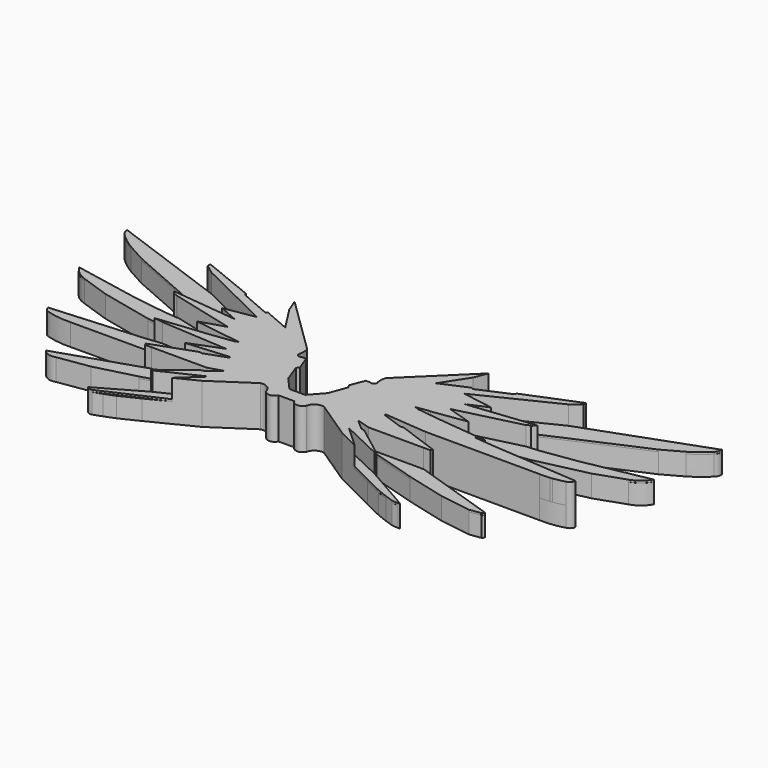
from build123d import *

# Parameters (mm, degrees)
F1_DEPTH = 5.08
F3_DEPTH = 0.508
F4_DEPTH = 5.334


# Not quite as in the source:
# - a feature names something its author has since deleted; it is built from what else it names


with BuildPart() as f1:
    # F0 (on Top) → F1 (new body)
    with BuildSketch(Plane.XY):
        with BuildLine():
            Line((-48.1556859188, 20.4166518488), (-45.7547713604, 18.6155719344))
            Line((-45.7547713604, 18.6155719344), (-76.2, 29.6858626598))
            ThreePointArc((-76.2, 29.6858626598), (-76.0861543316, 28.7560173531), (-75.5575876457, 27.9825896648))
            ThreePointArc((-75.5575876457, 27.9825896648), (-73.4489543022, 26.1296903536), (-71.1370066464, 24.5376889491))
            Line((-71.1370066464, 24.5376889491), (-66.2742528397, 21.8479481701))
            Line((-66.2742528397, 21.8479481701), (-58.5624668218, 18.4708371441))
            Line((-58.5624668218, 18.4708371441), (-35.3622883709, 8.3111182061))
            Line((-35.3622883709, 8.3111182061), (-29.5045119496, 5.7459068148))
            Line((-29.5045119496, 5.7459068148), (-46.2756385592, 7.5718067148))
            Line((-46.2756385592, 7.5718067148), (-46.5527664405, 7.6019780791))
            Line((-46.5527664405, 7.6019780791), (-45.7425475216, 6.6796372943))
            ThreePointArc((-45.7425475216, 6.6796372943), (-45.1421148672, 6.5863049394), (-44.6164082899, 6.2815708004))
            Line((-44.6164082899, 6.2815708004), (-48.1919185541, 6.5892115587))
            Line((-48.1919185541, 6.5892115587), (-57.1823799566, 7.911566844))
            Line((-57.1823799566, 7.911566844), (-73.6501002366, 11.0943052422))
            ThreePointArc((-73.6501002366, 11.0943052422), (-71.9881572625, 9.0822772608), (-69.6750634505, 7.8740107076))
            Line((-69.6750634505, 7.8740107076), (-62.2713321356, 5.3338180736))
            Line((-62.2713321356, 5.3338180736), (-48.9967867739, 2.3219788609))
            Line((-48.9967867739, 2.3219788609), (-26.0691300337, -1.000935792))
            Line((-26.0691300337, -1.000935792), (-25.5777875701, -1.000935792))
            Line((-25.5777875701, -1.000935792), (-22.5801609633, -1.4353830401))
            Line((-22.5801609633, -1.4353830401), (-23.598120873, -1.8208819811))
            Line((-23.598120873, -1.8208819811), (-29.6029133803, -2.5945054753))
            Line((-29.6029133803, -2.5945054753), (-42.3688777231, -3.9362549145))
            Line((-42.3688777231, -3.9362549145), (-40.0474588237, -4.2726991035))
            Line((-40.0474588237, -4.2726991035), (-44.609626805, -4.752199607))
            Line((-44.609626805, -4.752199607), (-67.5607632512, -6.4104881929))
            ThreePointArc((-67.5607632512, -6.4104881929), (-67.1610869389, -7.3442465842), (-66.2705799276, -7.8327577416))
            ThreePointArc((-66.2705799276, -7.8327577416), (-63.2022368013, -8.4748868798), (-60.0694551881, -8.5877528823))
            Line((-60.0694551881, -8.5877528823), (-30.8294042942, -8.5236300949))
            Line((-30.8294042942, -8.5236300949), (-19.9096897181, -7.6185828777))
            Line((-19.9096897181, -7.6185828777), (-19.9096897181, -7.9501351804))
            Line((-19.9096897181, -7.9501351804), (-25.3987332293, -9.9026141464))
            Line((-25.3987332293, -9.9026141464), (-26.177360162, -9.7897674271))
            Line((-26.177360162, -9.7897674271), (-36.7820497354, -13.6233741381))
            Line((-36.7820497354, -13.6233741381), (-36.5863546909, -14.1647142792))
            Line((-36.5863546909, -14.1647142792), (-34.8660396089, -14.1609416661))
            Line((-34.8660396089, -14.1609416661), (-56.2699958177, -21.2122522245))
            ThreePointArc((-56.2699958177, -21.2122522245), (-54.7449311758, -22.2892299122), (-52.8788538396, -22.2304210928))
            Line((-52.8788538396, -22.2304210928), (-44.9235154086, -21.0280555311))
            Line((-44.9235154086, -21.0280555311), (-34.6822151602, -18.375633369))
            Line((-34.6822151602, -18.375633369), (-17.2204277187, -13.107625142))
            Line((-17.2204277187, -13.107625142), (-19.9096897181, -15.4653348387))
            Line((-19.9096897181, -15.4653348387), (-20.953229799, -15.7801581493))
            Line((-20.953229799, -15.7801581493), (-28.8616205932, -21.8016796487))
            Line((-28.8616205932, -21.8016796487), (-28.4234154154, -21.865188904))
            Line((-28.4234154154, -21.865188904), (-39.7813339224, -28.3391517425))
            ThreePointArc((-39.7813339224, -28.3391517425), (-39.1733915256, -28.7871689471), (-38.4182988766, -28.7749843229))
            Line((-38.4182988766, -28.7749843229), (-36.202970226, -27.9869813522))
            Line((-36.202970226, -27.9869813522), (-33.5857428013, -26.9761213966))
            Line((-33.5857428013, -26.9761213966), (-28.8616205932, -24.6837501383))
            Line((-28.8616205932, -24.6837501383), (-17.9108938238, -19.2006514725))
            Line((-17.9108938238, -19.2006514725), (-8.1309387585, -12.6873564961))
            ThreePointArc((-8.1309387585, -12.6873564961), (-6.2540728234, -13.0090484092), (-5.155673966, -14.5645648429))
            ThreePointArc((-5.155673966, -14.5645648429), (-3.5896736899, -15.5530124109), (-2.0236734137, -14.5645648429))
            Line((-2.0236734137, -14.5645648429), (-2.0236734137, -12.7489120778))
            Line((-2.0236734137, -12.7489120778), (-2.0236734137, -11.069433426))
            Line((-2.0236734137, -11.069433426), (-5.0648916394, -7.6650855824))
            Line((-5.0648916394, -7.6650855824), (-6.7443696679, -3.1259542931))
            Line((-6.7443696679, -3.1259542931), (-6.245065625, -2.3543018679))
            Line((-6.245065625, -2.3543018679), (-7.6521960504, 1.2770033506))
            Line((-7.6521960504, 1.2770033506), (-8.7869788728, 1.2770033506))
            ThreePointArc((-8.7869788728, 1.2770033506), (-9.7426169592, 1.3351185179), (-9.9217616951, 2.2756123714))
            ThreePointArc((-9.9217616951, 2.2756123714), (-9.8496747918, 3.482472458), (-10.0676489398, 4.6716717941))
            Line((-10.0676489398, 4.6716717941), (-24.8806389617, 19.145210523))
            Line((-24.8806389617, 19.145210523), (-23.5544247636, 15.7928414245))
            Line((-23.5544247636, 15.7928414245), (-19.3413656313, 9.2291376834))
            Line((-19.3413656313, 9.2291376834), (-26.048319795, 12.124898042))
            Line((-26.048319795, 12.124898042), (-26.5740321425, 11.8401364598))
            Line((-26.5740321425, 11.8401364598), (-34.4378306482, 15.2353700376))
            Line((-34.4378306482, 15.2353700376), (-34.7242604777, 15.8157629926))
            Line((-34.7242604777, 15.8157629926), (-48.1556859188, 21.2768864279))
            ThreePointArc((-48.1556859188, 21.2768864279), (-48.1868505375, 20.8467691383), (-48.1556859188, 20.4166518488))
        make_face()
        with BuildLine():
            Line((5.0648916394, -7.6650855824), (2.0236734137, -11.069433426))
            Line((2.0236734137, -11.069433426), (2.0236734137, -12.7489120778))
            Line((2.0236734137, -12.7489120778), (2.0236734137, -14.5645648429))
            ThreePointArc((2.0236734137, -14.5645648429), (3.5896736899, -15.5530124109), (5.155673966, -14.5645648429))
            ThreePointArc((5.155673966, -14.5645648429), (6.2540728234, -13.0090484092), (8.1309387585, -12.6873564961))
            Line((8.1309387585, -12.6873564961), (17.9108938238, -19.2006514725))
            Line((17.9108938238, -19.2006514725), (28.8616205932, -24.6837501383))
            Line((28.8616205932, -24.6837501383), (33.5857428013, -26.9761213966))
            Line((33.5857428013, -26.9761213966), (36.202970226, -27.9869813522))
            Line((36.202970226, -27.9869813522), (38.4182988766, -28.7749843229))
            Line((38.4182988766, -28.7749843229), (40.0311607156, -28.87518605))
            Line((40.0311607156, -28.87518605), (40.5213075722, -28.804148866))
            Line((40.5213075722, -28.804148866), (39.7813339224, -28.3391517425))
            Line((39.7813339224, -28.3391517425), (28.4234154154, -21.865188904))
            Line((28.4234154154, -21.865188904), (28.8616205932, -21.8016796487))
            Line((28.8616205932, -21.8016796487), (20.953229799, -15.7801581493))
            Line((20.953229799, -15.7801581493), (19.9096897181, -15.4653348387))
            Line((19.9096897181, -15.4653348387), (17.2204277187, -13.107625142))
            Line((17.2204277187, -13.107625142), (34.6822151602, -18.375633369))
            Line((34.6822151602, -18.375633369), (44.9235154086, -21.0280555311))
            Line((44.9235154086, -21.0280555311), (52.8788538396, -22.2304210928))
            Line((52.8788538396, -22.2304210928), (55.8378268792, -21.801575922))
            Line((55.8378268792, -21.801575922), (56.2699958177, -21.2122522245))
            Line((56.2699958177, -21.2122522245), (34.8660396089, -14.1609416661))
            Line((34.8660396089, -14.1609416661), (36.5863546909, -14.1647142792))
            Line((36.5863546909, -14.1647142792), (36.7820497354, -13.6233741381))
            Line((36.7820497354, -13.6233741381), (26.177360162, -9.7897674271))
            Line((26.177360162, -9.7897674271), (25.3987332293, -9.9026141464))
            Line((25.3987332293, -9.9026141464), (19.9096897181, -7.9501351804))
            Line((19.9096897181, -7.9501351804), (19.9096897181, -7.6185828777))
            Line((19.9096897181, -7.6185828777), (30.8294042942, -8.5236300949))
            Line((30.8294042942, -8.5236300949), (60.0694551881, -8.5877528823))
            ThreePointArc((60.0694551881, -8.5877528823), (63.2022368013, -8.4748868798), (66.2705799276, -7.8327577416))
            ThreePointArc((66.2705799276, -7.8327577416), (67.1610869389, -7.3442465842), (67.5607632512, -6.4104881929))
            Line((67.5607632512, -6.4104881929), (44.609626805, -4.752199607))
            Line((44.609626805, -4.752199607), (40.0474588237, -4.2726991035))
            Line((40.0474588237, -4.2726991035), (42.3688777231, -3.9362549145))
            Line((42.3688777231, -3.9362549145), (29.6029133803, -2.5945054753))
            Line((29.6029133803, -2.5945054753), (23.598120873, -1.8208819811))
            Line((23.598120873, -1.8208819811), (22.5801609633, -1.4353830401))
            Line((22.5801609633, -1.4353830401), (25.5777875701, -1.000935792))
            Line((25.5777875701, -1.000935792), (26.0691300337, -1.000935792))
            Line((26.0691300337, -1.000935792), (48.9967867739, 2.3219788609))
            Line((48.9967867739, 2.3219788609), (62.2713321356, 5.3338180736))
            Line((62.2713321356, 5.3338180736), (69.6750634505, 7.8740107076))
            ThreePointArc((69.6750634505, 7.8740107076), (71.9881572625, 9.0822772608), (73.6501002366, 11.0943052422))
            Line((73.6501002366, 11.0943052422), (57.1823799566, 7.911566844))
            Line((57.1823799566, 7.911566844), (48.1919185541, 6.5892115587))
            Line((48.1919185541, 6.5892115587), (44.6164082899, 6.2815708004))
            ThreePointArc((44.6164082899, 6.2815708004), (45.1421148672, 6.5863049394), (45.7425475216, 6.6796372943))
            Line((45.7425475216, 6.6796372943), (46.5527664405, 7.6019780791))
            Line((46.5527664405, 7.6019780791), (46.2756385592, 7.5718067148))
            Line((46.2756385592, 7.5718067148), (29.5045119496, 5.7459068148))
            Line((29.5045119496, 5.7459068148), (35.3622883709, 8.3111182061))
            Line((35.3622883709, 8.3111182061), (58.5624668218, 18.4708371441))
            Line((58.5624668218, 18.4708371441), (66.2742528397, 21.8479481701))
            Line((66.2742528397, 21.8479481701), (71.1370066464, 24.5376889491))
            ThreePointArc((71.1370066464, 24.5376889491), (73.4489543022, 26.1296903536), (75.5575876457, 27.9825896648))
            ThreePointArc((75.5575876457, 27.9825896648), (76.0861543316, 28.7560173531), (76.2, 29.6858626598))
            Line((76.2, 29.6858626598), (45.7547713604, 18.6155719344))
            Line((45.7547713604, 18.6155719344), (48.1556859188, 20.4166518488))
            ThreePointArc((48.1556859188, 20.4166518488), (48.1868505375, 20.8467691383), (48.1556859188, 21.2768864279))
            Line((48.1556859188, 21.2768864279), (34.7242604777, 15.8157629926))
            Line((34.7242604777, 15.8157629926), (34.4378306482, 15.2353700376))
            Line((34.4378306482, 15.2353700376), (26.5740321425, 11.8401364598))
            Line((26.5740321425, 11.8401364598), (26.048319795, 12.124898042))
            Line((26.048319795, 12.124898042), (19.3413656313, 9.2291376834))
            Line((19.3413656313, 9.2291376834), (23.5544247636, 15.7928414245))
            Line((23.5544247636, 15.7928414245), (24.8806389617, 19.145210523))
            Line((24.8806389617, 19.145210523), (10.0676489398, 4.6716717941))
            ThreePointArc((10.0676489398, 4.6716717941), (9.8496747918, 3.482472458), (9.9217616951, 2.2756123714))
            ThreePointArc((9.9217616951, 2.2756123714), (9.7426169592, 1.3351185179), (8.7869788728, 1.2770033506))
            Line((8.7869788728, 1.2770033506), (7.6521960504, 1.2770033506))
            Line((7.6521960504, 1.2770033506), (6.245065625, -2.3543018679))
            Line((6.245065625, -2.3543018679), (6.7443696679, -3.1259542931))
            Line((6.7443696679, -3.1259542931), (5.0648916394, -7.6650855824))
        make_face()
        Polygon((2.0236734137, -11.069433426), (-2.0236734137, -11.069433426), (-2.0236734137, -12.7489120778), (-2.0236734137, -14.5645648429), (2.0236734137, -14.5645648429), (2.0236734137, -12.7489120778), align=None)
    extrude(amount=F1_DEPTH)

    # F2 (on face) → F3 (join)
    with BuildSketch(Plane.XY.offset(5.08)):
        with BuildLine():
            Line((-45.7547713604, 18.6155719344), (-76.2, 29.6858626598))
            ThreePointArc((-76.2, 29.6858626598), (-76.0613798938, 28.8812729633), (-75.7155257761, 28.1417021128))
            ThreePointArc((-75.7155257761, 28.1417021128), (-75.6388106018, 28.0599086326), (-75.5575876457, 27.9825896648))
            ThreePointArc((-75.5575876457, 27.9825896648), (-75.1114300748, 27.5526583841), (-74.6542423004, 27.1344756214))
            ThreePointArc((-74.6542423004, 27.1344756214), (-72.9553220799, 25.7552244495), (-71.1370066464, 24.5376889491))
            Line((-71.1370066464, 24.5376889491), (-66.2742528397, 21.8479481701))
            Line((-66.2742528397, 21.8479481701), (-34.4378306482, 7.9062837928))
            Line((-34.4378306482, 7.9062837928), (-26.5740321425, 9.2291376834))
            Line((-26.5740321425, 9.2291376834), (-45.7547713604, 18.6155719344))
        make_face()
        with BuildLine():
            Line((-57.1823799566, 7.911566844), (-73.6501002366, 11.0943052422))
            ThreePointArc((-73.6501002366, 11.0943052422), (-71.9475816852, 9.1323625591), (-69.6750634505, 7.8740107076))
            Line((-69.6750634505, 7.8740107076), (-62.2713321356, 5.3338180736))
            Line((-62.2713321356, 5.3338180736), (-48.9967867739, 2.3219788609))
            Line((-48.9967867739, 2.3219788609), (-34.8303394704, 0.2688298689))
            Line((-34.8303394704, 0.2688298689), (-28.4082200378, 2.2570914589))
            Line((-28.4082200378, 2.2570914589), (-44.8570793006, 6.4537258018))
            ThreePointArc((-44.8570793006, 6.4537258018), (-44.7328690892, 6.3730651023), (-44.6164082899, 6.2815708004))
            Line((-44.6164082899, 6.2815708004), (-48.1919185541, 6.5892115587))
            Line((-48.1919185541, 6.5892115587), (-57.1823799566, 7.911566844))
        make_face()
        with BuildLine():
            Line((-22.8044074029, -5.3703207523), (-40.0474588237, -4.2726991035))
            Line((-40.0474588237, -4.2726991035), (-44.609626805, -4.752199607))
            Line((-44.609626805, -4.752199607), (-67.5607632512, -6.4104881929))
            ThreePointArc((-67.5607632512, -6.4104881929), (-67.1610869389, -7.3442465842), (-66.2705799276, -7.8327577416))
            ThreePointArc((-66.2705799276, -7.8327577416), (-63.2022368013, -8.4748868798), (-60.0694551881, -8.5877528823))
            Line((-60.0694551881, -8.5877528823), (-30.8294042942, -8.5236300949))
            Line((-30.8294042942, -8.5236300949), (-22.8044074029, -5.3703207523))
        make_face()
        with BuildLine():
            Line((-20.7118401198, -14.1609416661), (-34.8660396089, -14.1609416661))
            Line((-34.8660396089, -14.1609416661), (-56.2699958177, -21.2122522245))
            ThreePointArc((-56.2699958177, -21.2122522245), (-54.7449311758, -22.2892299122), (-52.8788538396, -22.2304210928))
            Line((-52.8788538396, -22.2304210928), (-44.9235154086, -21.0280555311))
            Line((-44.9235154086, -21.0280555311), (-34.6822151602, -18.375633369))
            Line((-34.6822151602, -18.375633369), (-20.7118401198, -14.1609416661))
        make_face()
        with BuildLine():
            Line((-17.9108938238, -16.889270395), (-28.4234154154, -21.865188904))
            Line((-28.4234154154, -21.865188904), (-29.785812622, -22.641749229))
            Line((-29.785812622, -22.641749229), (-39.7813339224, -28.3391517425))
            ThreePointArc((-39.7813339224, -28.3391517425), (-39.1733915256, -28.7871689471), (-38.4182988766, -28.7749843229))
            Line((-38.4182988766, -28.7749843229), (-23.3862572085, -21.9422008054))
            Line((-23.3862572085, -21.9422008054), (-17.9108938238, -16.889270395))
        make_face()
        with BuildLine():
            Line((76.2, 29.6858626598), (45.7547713604, 18.6155719344))
            Line((45.7547713604, 18.6155719344), (26.5740321425, 9.2291376834))
            Line((26.5740321425, 9.2291376834), (34.4378306482, 7.9062837928))
            Line((34.4378306482, 7.9062837928), (66.2742528397, 21.8479481701))
            Line((66.2742528397, 21.8479481701), (71.1370066464, 24.5376889491))
            ThreePointArc((71.1370066464, 24.5376889491), (72.9553220799, 25.7552244495), (74.6542423004, 27.1344756214))
            ThreePointArc((74.6542423004, 27.1344756214), (75.1114300748, 27.5526583841), (75.5575876457, 27.9825896648))
            ThreePointArc((75.5575876457, 27.9825896648), (75.6388106018, 28.0599086326), (75.7155257761, 28.1417021128))
            ThreePointArc((75.7155257761, 28.1417021128), (76.0613798938, 28.8812729633), (76.2, 29.6858626598))
        make_face()
        with BuildLine():
            Line((17.9108938238, -16.889270395), (23.3862572085, -21.9422008054))
            Line((23.3862572085, -21.9422008054), (29.4455388981, -24.967095378))
            Line((29.4455388981, -24.967095378), (32.5631852092, -26.4799272825))
            Line((32.5631852092, -26.4799272825), (35.1217063863, -27.5693614287))
            Line((35.1217063863, -27.5693614287), (36.202970226, -27.9869813522))
            Line((36.202970226, -27.9869813522), (38.4182988766, -28.7749843229))
            ThreePointArc((38.4182988766, -28.7749843229), (39.0234464973, -28.8015241098), (39.627225653, -28.8500909117))
            Line((39.627225653, -28.8500909117), (40.0311607156, -28.87518605))
            Line((40.0311607156, -28.87518605), (40.5213075722, -28.804148866))
            Line((40.5213075722, -28.804148866), (39.7813339224, -28.3391517425))
            Line((39.7813339224, -28.3391517425), (28.4234154154, -21.865188904))
            Line((28.4234154154, -21.865188904), (17.9108938238, -16.889270395))
        make_face()
        with BuildLine():
            Line((48.1919185541, 6.5892115587), (44.6545333062, 6.284851118))
            Line((44.6545333062, 6.284851118), (28.4082200378, 2.2570914589))
            Line((28.4082200378, 2.2570914589), (34.8303394704, 0.2688298689))
            Line((34.8303394704, 0.2688298689), (48.9967867739, 2.3219788609))
            Line((48.9967867739, 2.3219788609), (62.2713321356, 5.3338180736))
            Line((62.2713321356, 5.3338180736), (69.6750634505, 7.8740107076))
            ThreePointArc((69.6750634505, 7.8740107076), (71.9475816852, 9.1323625591), (73.6501002366, 11.0943052422))
            Line((73.6501002366, 11.0943052422), (57.1823799566, 7.911566844))
            Line((57.1823799566, 7.911566844), (48.1919185541, 6.5892115587))
        make_face()
        with BuildLine():
            Line((34.8660396089, -14.1609416661), (20.7118401198, -14.1609416661))
            Line((20.7118401198, -14.1609416661), (34.6822151602, -18.375633369))
            Line((34.6822151602, -18.375633369), (44.9235154086, -21.0280555311))
            Line((44.9235154086, -21.0280555311), (52.8788538396, -22.2304210928))
            Line((52.8788538396, -22.2304210928), (55.6730115418, -21.8254626761))
            ThreePointArc((55.6730115418, -21.8254626761), (55.9941957529, -21.540949068), (56.2699958177, -21.2122522245))
            Line((56.2699958177, -21.2122522245), (34.8660396089, -14.1609416661))
        make_face()
        with BuildLine():
            Line((44.609626805, -4.752199607), (40.0474588237, -4.2726991035))
            Line((40.0474588237, -4.2726991035), (22.8044074029, -5.3703207523))
            Line((22.8044074029, -5.3703207523), (30.8294042942, -8.5236300949))
            Line((30.8294042942, -8.5236300949), (62.7568216743, -8.5236300949))
            ThreePointArc((62.7568216743, -8.5236300949), (63.0066080535, -8.4976449239), (63.2560171957, -8.4682588034))
            Line((63.2560171957, -8.4682588034), (65.3207376599, -8.0048982054))
            ThreePointArc((65.3207376599, -8.0048982054), (66.6014512665, -7.4334656957), (67.5607632512, -6.4104881929))
            Line((67.5607632512, -6.4104881929), (44.609626805, -4.752199607))
        make_face()
        Polygon((67.5607632512, -6.4104881929), (40.0474588237, -4.2726991035), (44.609626805, -4.752199607), align=None)
        with BuildLine():
            ThreePointArc((66.2705799276, -7.8327577416), (67.1610869389, -7.3442465842), (67.5607632512, -6.4104881929))
            ThreePointArc((67.5607632512, -6.4104881929), (66.6014512665, -7.4334656957), (65.3207376599, -8.0048982054))
            Line((65.3207376599, -8.0048982054), (63.2560171957, -8.4682588034))
            ThreePointArc((63.2560171957, -8.4682588034), (64.7765999277, -8.2136046301), (66.2705799276, -7.8327577416))
        make_face()
        with BuildLine():
            Line((62.7568216743, -8.5236300949), (30.8294042942, -8.5236300949))
            Line((30.8294042942, -8.5236300949), (60.0694551881, -8.5877528823))
            ThreePointArc((60.0694551881, -8.5877528823), (61.414308994, -8.604749419), (62.7568216743, -8.5236300949))
        make_face()
    extrude(amount=F3_DEPTH)

    # F2 (on face) → F4 (join)
    with BuildSketch(Plane.XY.offset(5.08)):
        with BuildLine():
            Line((-48.1556859188, 20.4166518488), (-45.7547713604, 18.6155719344))
            Line((-45.7547713604, 18.6155719344), (-26.5740321425, 9.2291376834))
            Line((-26.5740321425, 9.2291376834), (-34.4378306482, 7.9062837928))
            Line((-34.4378306482, 7.9062837928), (-29.5045119496, 5.7459068148))
            Line((-29.5045119496, 5.7459068148), (-46.5527664405, 7.6019780791))
            Line((-46.5527664405, 7.6019780791), (-45.7425475216, 6.6796372943))
            ThreePointArc((-45.7425475216, 6.6796372943), (-45.2838287455, 6.6293340197), (-44.8570793006, 6.4537258018))
            Line((-44.8570793006, 6.4537258018), (-28.4082200378, 2.2570914589))
            Line((-28.4082200378, 2.2570914589), (-34.8303394704, 0.2688298689))
            Line((-34.8303394704, 0.2688298689), (-26.0691300337, -1.000935792))
            Line((-26.0691300337, -1.000935792), (-25.5777875701, -1.000935792))
            Line((-25.5777875701, -1.000935792), (-22.5801609633, -1.4353830401))
            Line((-22.5801609633, -1.4353830401), (-23.598120873, -1.8208819811))
            Line((-23.598120873, -1.8208819811), (-29.6029133803, -2.5945054753))
            Line((-29.6029133803, -2.5945054753), (-42.3688777231, -3.9362549145))
            Line((-42.3688777231, -3.9362549145), (-40.0474588237, -4.2726991035))
            Line((-40.0474588237, -4.2726991035), (-22.8044074029, -5.3703207523))
            Line((-22.8044074029, -5.3703207523), (-30.8294042942, -8.5236300949))
            Line((-30.8294042942, -8.5236300949), (-19.9096897181, -7.6185828777))
            Line((-19.9096897181, -7.6185828777), (-19.9096897181, -7.9501351804))
            Line((-19.9096897181, -7.9501351804), (-25.3987332293, -9.9026141464))
            Line((-25.3987332293, -9.9026141464), (-26.177360162, -9.7897674271))
            Line((-26.177360162, -9.7897674271), (-36.7820497354, -13.6233741381))
            Line((-36.7820497354, -13.6233741381), (-36.5863546909, -14.1647142792))
            Line((-36.5863546909, -14.1647142792), (-34.8660396089, -14.1609416661))
            Line((-34.8660396089, -14.1609416661), (-20.7118401198, -14.1609416661))
            Line((-20.7118401198, -14.1609416661), (-17.2204277187, -13.107625142))
            Line((-17.2204277187, -13.107625142), (-19.9096897181, -15.4653348387))
            Line((-19.9096897181, -15.4653348387), (-20.953229799, -15.7801581493))
            Line((-20.953229799, -15.7801581493), (-28.8616205932, -21.8016796487))
            Line((-28.8616205932, -21.8016796487), (-28.4234154154, -21.865188904))
            Line((-28.4234154154, -21.865188904), (-17.9108938238, -16.889270395))
            Line((-17.9108938238, -16.889270395), (-23.3862572085, -21.9422008054))
            Line((-23.3862572085, -21.9422008054), (-17.9108938238, -19.2006514725))
            Line((-17.9108938238, -19.2006514725), (-8.1309387585, -12.6873564961))
            ThreePointArc((-8.1309387585, -12.6873564961), (-6.2540728234, -13.0090484092), (-5.155673966, -14.5645648429))
            ThreePointArc((-5.155673966, -14.5645648429), (-3.5896736899, -15.5530124109), (-2.0236734137, -14.5645648429))
            Line((-2.0236734137, -14.5645648429), (2.0236734137, -14.5645648429))
            ThreePointArc((2.0236734137, -14.5645648429), (3.5896736899, -15.5530124109), (5.155673966, -14.5645648429))
            ThreePointArc((5.155673966, -14.5645648429), (6.2540728234, -13.0090484092), (8.1309387585, -12.6873564961))
            Line((8.1309387585, -12.6873564961), (17.9108938238, -19.2006514725))
            Line((17.9108938238, -19.2006514725), (23.3862572085, -21.9422008054))
            Line((23.3862572085, -21.9422008054), (17.9108938238, -16.889270395))
            Line((17.9108938238, -16.889270395), (28.4234154154, -21.865188904))
            Line((28.4234154154, -21.865188904), (28.8616205932, -21.8016796487))
            Line((28.8616205932, -21.8016796487), (20.953229799, -15.7801581493))
            Line((20.953229799, -15.7801581493), (19.9096897181, -15.4653348387))
            Line((19.9096897181, -15.4653348387), (17.2204277187, -13.107625142))
            Line((17.2204277187, -13.107625142), (20.7118401198, -14.1609416661))
            Line((20.7118401198, -14.1609416661), (34.8660396089, -14.1609416661))
            Line((34.8660396089, -14.1609416661), (36.5863546909, -14.1647142792))
            Line((36.5863546909, -14.1647142792), (36.7820497354, -13.6233741381))
            Line((36.7820497354, -13.6233741381), (26.177360162, -9.7897674271))
            Line((26.177360162, -9.7897674271), (25.3987332293, -9.9026141464))
            Line((25.3987332293, -9.9026141464), (19.9096897181, -7.9501351804))
            Line((19.9096897181, -7.9501351804), (19.9096897181, -7.6185828777))
            Line((19.9096897181, -7.6185828777), (30.8294042942, -8.5236300949))
            Line((30.8294042942, -8.5236300949), (22.8044074029, -5.3703207523))
            Line((22.8044074029, -5.3703207523), (40.0474588237, -4.2726991035))
            Line((40.0474588237, -4.2726991035), (42.3688777231, -3.9362549145))
            Line((42.3688777231, -3.9362549145), (29.6029133803, -2.5945054753))
            Line((29.6029133803, -2.5945054753), (23.598120873, -1.8208819811))
            Line((23.598120873, -1.8208819811), (22.5801609633, -1.4353830401))
            Line((22.5801609633, -1.4353830401), (25.5777875701, -1.000935792))
            Line((25.5777875701, -1.000935792), (26.0691300337, -1.000935792))
            Line((26.0691300337, -1.000935792), (34.8303394704, 0.2688298689))
            Line((34.8303394704, 0.2688298689), (28.4082200378, 2.2570914589))
            Line((28.4082200378, 2.2570914589), (44.6545333062, 6.284851118))
            Line((44.6545333062, 6.284851118), (44.6164082899, 6.2815708004))
            ThreePointArc((44.6164082899, 6.2815708004), (45.1421148672, 6.5863049394), (45.7425475216, 6.6796372943))
            Line((45.7425475216, 6.6796372943), (46.5527664405, 7.6019780791))
            Line((46.5527664405, 7.6019780791), (29.5045119496, 5.7459068148))
            Line((29.5045119496, 5.7459068148), (34.4378306482, 7.9062837928))
            Line((34.4378306482, 7.9062837928), (26.5740321425, 9.2291376834))
            Line((26.5740321425, 9.2291376834), (45.7547713604, 18.6155719344))
            Line((45.7547713604, 18.6155719344), (48.1556859188, 20.4166518488))
            ThreePointArc((48.1556859188, 20.4166518488), (48.1868505375, 20.8467691383), (48.1556859188, 21.2768864279))
            Line((48.1556859188, 21.2768864279), (34.7242604777, 15.8157629926))
            Line((34.7242604777, 15.8157629926), (34.4378306482, 15.2353700376))
            Line((34.4378306482, 15.2353700376), (26.5740321425, 11.8401364598))
            Line((26.5740321425, 11.8401364598), (26.048319795, 12.124898042))
            Line((26.048319795, 12.124898042), (19.3413656313, 9.2291376834))
            Line((19.3413656313, 9.2291376834), (23.5544247636, 15.7928414245))
            Line((23.5544247636, 15.7928414245), (24.8806389617, 19.145210523))
            Line((24.8806389617, 19.145210523), (10.0676489398, 4.6716717941))
            ThreePointArc((10.0676489398, 4.6716717941), (9.8496747918, 3.482472458), (9.9217616951, 2.2756123714))
            ThreePointArc((9.9217616951, 2.2756123714), (9.7426169592, 1.3351185179), (8.7869788728, 1.2770033506))
            Line((8.7869788728, 1.2770033506), (7.6521960504, 1.2770033506))
            Line((7.6521960504, 1.2770033506), (6.245065625, -2.3543018679))
            Line((6.245065625, -2.3543018679), (6.7443696679, -3.1259542931))
            Line((6.7443696679, -3.1259542931), (5.0648916394, -7.6650855824))
            Line((5.0648916394, -7.6650855824), (2.0236734137, -11.069433426))
            Line((2.0236734137, -11.069433426), (-2.0236734137, -11.069433426))
            Line((-2.0236734137, -11.069433426), (-5.0648916394, -7.6650855824))
            Line((-5.0648916394, -7.6650855824), (-6.7443696679, -3.1259542931))
            Line((-6.7443696679, -3.1259542931), (-6.245065625, -2.3543018679))
            Line((-6.245065625, -2.3543018679), (-7.6521960504, 1.2770033506))
            Line((-7.6521960504, 1.2770033506), (-8.7869788728, 1.2770033506))
            ThreePointArc((-8.7869788728, 1.2770033506), (-9.7426169592, 1.3351185179), (-9.9217616951, 2.2756123714))
            ThreePointArc((-9.9217616951, 2.2756123714), (-9.8496747918, 3.482472458), (-10.0676489398, 4.6716717941))
            Line((-10.0676489398, 4.6716717941), (-24.8806389617, 19.145210523))
            Line((-24.8806389617, 19.145210523), (-23.5544247636, 15.7928414245))
            Line((-23.5544247636, 15.7928414245), (-19.3413656313, 9.2291376834))
            Line((-19.3413656313, 9.2291376834), (-26.048319795, 12.124898042))
            Line((-26.048319795, 12.124898042), (-26.5740321425, 11.8401364598))
            Line((-26.5740321425, 11.8401364598), (-34.4378306482, 15.2353700376))
            Line((-34.4378306482, 15.2353700376), (-34.7242604777, 15.8157629926))
            Line((-34.7242604777, 15.8157629926), (-48.1556859188, 21.2768864279))
            ThreePointArc((-48.1556859188, 21.2768864279), (-48.1868505375, 20.8467691383), (-48.1556859188, 20.4166518488))
        make_face()
        with BuildLine():
            Line((44.609626805, -4.752199607), (40.0474588237, -4.2726991035))
            Line((40.0474588237, -4.2726991035), (22.8044074029, -5.3703207523))
            Line((22.8044074029, -5.3703207523), (30.8294042942, -8.5236300949))
            Line((30.8294042942, -8.5236300949), (62.7568216743, -8.5236300949))
            ThreePointArc((62.7568216743, -8.5236300949), (63.0066080535, -8.4976449239), (63.2560171957, -8.4682588034))
            Line((63.2560171957, -8.4682588034), (65.3207376599, -8.0048982054))
            ThreePointArc((65.3207376599, -8.0048982054), (66.6014512665, -7.4334656957), (67.5607632512, -6.4104881929))
            Line((67.5607632512, -6.4104881929), (44.609626805, -4.752199607))
        make_face()
        with BuildLine():
            ThreePointArc((66.2705799276, -7.8327577416), (67.1610869389, -7.3442465842), (67.5607632512, -6.4104881929))
            ThreePointArc((67.5607632512, -6.4104881929), (66.6014512665, -7.4334656957), (65.3207376599, -8.0048982054))
            Line((65.3207376599, -8.0048982054), (63.2560171957, -8.4682588034))
            ThreePointArc((63.2560171957, -8.4682588034), (64.7765999277, -8.2136046301), (66.2705799276, -7.8327577416))
        make_face()
        with BuildLine():
            Line((62.7568216743, -8.5236300949), (30.8294042942, -8.5236300949))
            Line((30.8294042942, -8.5236300949), (60.0694551881, -8.5877528823))
            ThreePointArc((60.0694551881, -8.5877528823), (61.414308994, -8.604749419), (62.7568216743, -8.5236300949))
        make_face()
    extrude(amount=F4_DEPTH)


solid = f1.part
